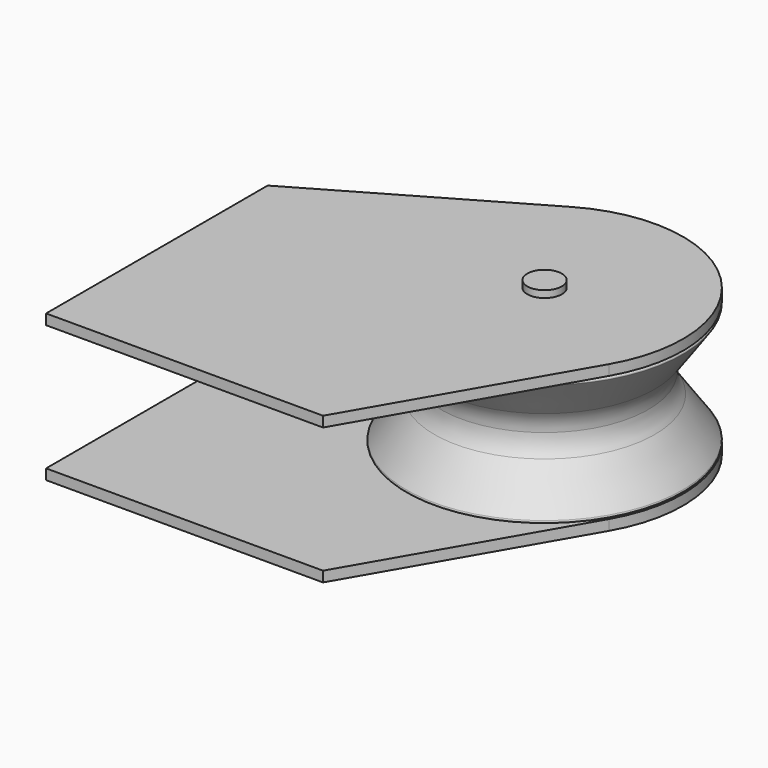
from build123d import *
from build123d import SkipClean  # not in build123d's __all__

# Parameters (mm, degrees)
F0_W     = 25
F0_H     = 10
F0_H_2   = 15
F0_W_2   = 175
F5_DEPTH = 15


# Not quite as in the source:
# - ends of sketch curves that miss each other by under 0.0002 mm in the source are joined


with BuildPart() as f1:
    # F0 (on Right) → F1 (revolve)
    with BuildSketch(Plane.YZ):
        with Locations((12.5, 111)):
            Rectangle(F0_W, F0_H)
        with Locations((12.5, 98.5)):
            Rectangle(F0_W, F0_H_2)
        Polygon((0, 0), (25, 0), (25, 90), (25, 91), (0, 91), align=None)
    revolve(axis=Axis((0, 0, 58), (0, 0, 1)))

    # F0 (on Right) → F2 (revolve)
    with BuildSketch(Plane.YZ):
        with BuildLine():
            ThreePointArc((150, 0), (152.3425507406, 15.1250629778), (159.1507012033, 28.8328768565))
            Line((159.1507012033, 28.8328768565), (199.542465, 86.058356))
            ThreePointArc((199.542465, 86.058356), (199.7196970287, 88.6501935058), (197.5, 90))
            Line((197.5, 90), (25, 90))
            Line((25, 90), (25, 0))
            Line((25, 0), (150, 0))
        make_face()
    revolve(axis=Axis((0, 0, 58), (0, 0, 1)))

    # F0 (on Right) → F3 (revolve)
    with BuildSketch(Plane.YZ):
        with Locations((112.5, 98.5)):
            Rectangle(F0_W_2, F0_H_2)
    revolve(axis=Axis((0, 0, 58), (0, 0, 1)))

    # F4 (on face) → F5 (join, through all)
    with BuildSketch(Plane.XY.offset(106)):
        with BuildLine():
            ThreePointArc((0, -200), (-141.4213562373, -141.4213562373), (-200, 0))
            Line((-200, 0), (-400, 0))
            Line((-400, 0), (-400, -400))
            Line((-400, -400), (0, -400))
            Line((0, -400), (0, -200))
        make_face()
        with BuildLine():
            Line((-400, 0), (-200, 0))
            ThreePointArc((-200, 0), (-173.2050807569, 100), (-100, 173.2050807569))
            Line((-100, 173.2050807569), (-400, 0))
        make_face()
        with BuildLine():
            ThreePointArc((173.2050807569, -100), (100, -173.2050807569), (0, -200))
            Line((0, -200), (0, -400))
            Line((0, -400), (173.2050807569, -100))
        make_face()
    extrude(amount=-F5_DEPTH)

    # F6: F1 across face


with BuildPart() as f1_1:
    add(f1.part, clean=False)
    with SkipClean():  # cleaning this boolean's faces spoils the solid; the shape is the same uncleaned
        add(f1.part.mirror(Plane(origin=(0, 0, 0), x_dir=(1, 0, 0), z_dir=(0, 0, -1))), clean=False)


solid = f1_1.part
